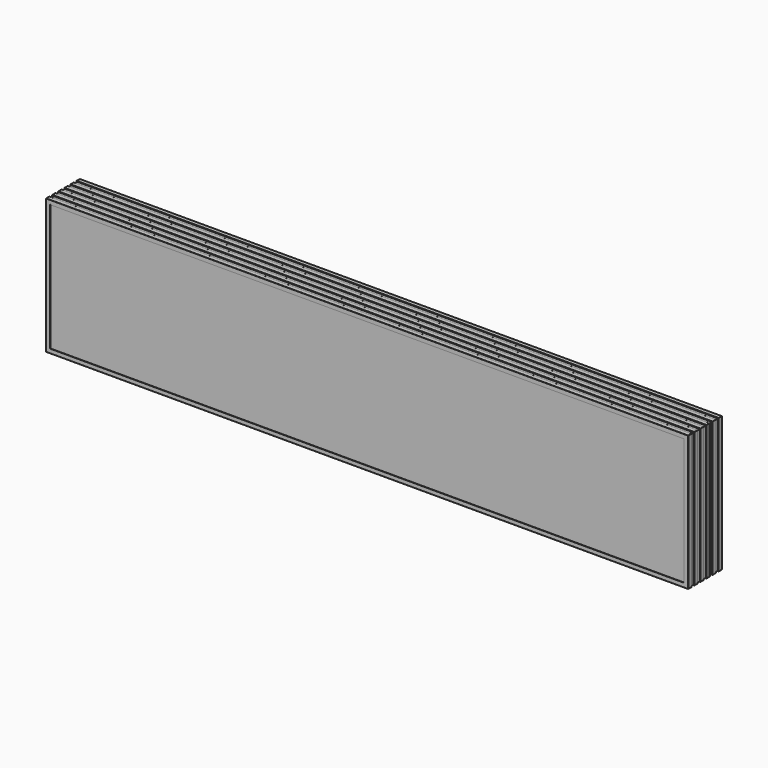
from build123d import *

# Parameters (mm, degrees)
F0_W      = 50
F0_H      = 2720
F1_DEPTH  = 100
F2_W      = 1520
F2_H      = 100
F3_DEPTH  = 320
F2_W_2    = 3000
F2_W_3    = 1220
F4_W      = 1500
F4_H      = 300
F4_W_2    = 2980
F4_W_3    = 1200
F5_DEPTH  = 100.001
F6_W      = 8
F6_H      = 1.5
F7_DEPTH  = 5840.001
F8_W      = 1.5
F8_H      = 8
F9_DEPTH  = 2720.001
F11_W     = 2980
F11_H     = 300
F12_DEPTH = 98
F11_W_2   = 1200
F11_W_3   = 1500
F13_R     = 0.5
F13_2_R   = 0.5
F13_3_R   = 0.5
F13_4_R   = 0.5


# Not quite as in the source:
# - two fillets or chamfers of one size are made in one step


with BuildPart() as f1:
    # F0 (on Front) → F1 (new body)
    with BuildSketch(Plane.XZ):
        with Locations((-1525, -1360)):
            Rectangle(F0_W, F0_H)
    extrude(amount=F1_DEPTH)


with BuildPart() as f1b:
    # F0 (on Front) → F1, piece 2 (new body)
    with BuildSketch(Plane.XZ):
        with Locations((1525, -1360)):
            Rectangle(F0_W, F0_H)
    extrude(amount=F1_DEPTH)


with BuildPart() as f3:
    # F2 (on face) → F3 (new body)
    with BuildSketch(Plane.XY):
        with Locations((-2310, -50)):
            Rectangle(F2_W, F2_H)
    extrude(amount=-F3_DEPTH)


with BuildPart() as f3b:
    # F2 (on face) → F3, piece 2 (new body)
    with BuildSketch(Plane.XY):
        with Locations((0, -50)):
            Rectangle(F2_W_2, F2_H)
    extrude(amount=-F3_DEPTH)


with BuildPart() as f3c:
    # F2 (on face) → F3, piece 3 (new body)
    with BuildSketch(Plane.XY):
        with Locations((2160, -50)):
            Rectangle(F2_W_3, F2_H)
    extrude(amount=-F3_DEPTH)


with BuildPart() as f5_tool:
    # F4 (on face) → F5 (new body, through all)
    with BuildSketch(Plane.XZ.offset(100)):
        with Locations((-2310, -160)):
            Rectangle(F4_W, F4_H)
        with Locations((0, -160)):
            Rectangle(F4_W_2, F4_H)
        with Locations((2160, -160)):
            Rectangle(F4_W_3, F4_H)
    extrude(amount=-F5_DEPTH)


with BuildPart() as f3_1:
    add(f3.part)

    # F5: cut by f5_tool
    add(f5_tool.part, mode=Mode.SUBTRACT)


with BuildPart() as f3b_1:
    add(f3b.part)

    # F5: cut by f5_tool
    add(f5_tool.part, mode=Mode.SUBTRACT)


with BuildPart() as f3c_1:
    add(f3c.part)

    # F5: cut by f5_tool
    add(f5_tool.part, mode=Mode.SUBTRACT)


with BuildPart() as f7_tool:
    # F6 (on face) → F7 (new body, through all)
    with BuildSketch(Plane(origin=(-3070, 0, 0), x_dir=(0, -1, 0), z_dir=(-1, 0, 0))):
        with Locations((14, -0.75)):
            Rectangle(F6_W, F6_H)
        with Locations((32, -0.75)):
            Rectangle(F6_W, F6_H)
        with Locations((50, -0.75)):
            Rectangle(F6_W, F6_H)
        with Locations((68, -0.75)):
            Rectangle(F6_W, F6_H)
        with Locations((86, -0.75)):
            Rectangle(F6_W, F6_H)
        with Locations((86, -319.25)):
            Rectangle(F6_W, F6_H)
        with Locations((68, -319.25)):
            Rectangle(F6_W, F6_H)
        with Locations((14, -319.25)):
            Rectangle(F6_W, F6_H)
        with Locations((32, -319.25)):
            Rectangle(F6_W, F6_H)
        with Locations((50, -319.25)):
            Rectangle(F6_W, F6_H)
    extrude(amount=-F7_DEPTH)


with BuildPart() as f1_1:
    add(f1.part)

    # F7: cut by f7_tool
    add(f7_tool.part, mode=Mode.SUBTRACT)


with BuildPart() as f1b_1:
    add(f1b.part)

    # F7: cut by f7_tool
    add(f7_tool.part, mode=Mode.SUBTRACT)

    # F13
    f13_edges = [f1b_1.edges().sort_by_distance(p)[0] for p in [
        (1525, -90, 0),
        (1525, -100, 0),
        (1525, -72, 0),
        (1525, -82, 0),
        (1525, -54, 0),
        (1525, -64, 0),
        (1525, -36, 0),
        (1525, -46, 0),
        (1525, -18, 0),
        (1525, -28, 0),
        (1525, 0, 0),
        (1525, -10, 0),
    ]]
    fillet(f13_edges, radius=F13_R)


with BuildPart() as f3_2:
    add(f3_1.part)

    # F7: cut by f7_tool
    add(f7_tool.part, mode=Mode.SUBTRACT)

    # F8 (on face) → F9 (cut, through all)
    with BuildSketch(Plane.XY):
        with Locations((-3069.25, -86)):
            Rectangle(F8_W, F8_H)
        with Locations((-3069.25, -68)):
            Rectangle(F8_W, F8_H)
        with Locations((-3069.25, -50)):
            Rectangle(F8_W, F8_H)
        with Locations((-3069.25, -32)):
            Rectangle(F8_W, F8_H)
        with Locations((-3069.25, -14)):
            Rectangle(F8_W, F8_H)
        with Locations((3069.25, -68)):
            Rectangle(F8_W, F8_H)
        with Locations((3069.25, -32)):
            Rectangle(F8_W, F8_H)
        with Locations((3069.25, -86)):
            Rectangle(F8_W, F8_H)
        with Locations((3069.25, -50)):
            Rectangle(F8_W, F8_H)
        with Locations((3069.25, -14)):
            Rectangle(F8_W, F8_H)
        with Locations((-1550.75, -86)):
            Rectangle(F8_W, F8_H)
        with Locations((-1550.75, -68)):
            Rectangle(F8_W, F8_H)
        with Locations((-1550.75, -50)):
            Rectangle(F8_W, F8_H)
        with Locations((-1550.75, -32)):
            Rectangle(F8_W, F8_H)
        with Locations((-1550.75, -14)):
            Rectangle(F8_W, F8_H)
    extrude(amount=-F9_DEPTH, mode=Mode.SUBTRACT)

    # F13#2
    f13_2_edges = [f3_2.edges().sort_by_distance(p)[0] for p in [
        (-1550, -5, -320),
        (-1550, -23, -320),
        (-1550, -41, -320),
        (-1550, -59, -320),
        (-1550, -77, -320),
        (-1550, -95, -320),
        (-3070, -95, -320),
        (-3068.5, -86, -318.5),
        (-3070, -77, -320),
        (-3068.5, -68, -318.5),
        (-3070, -59, -320),
        (-3068.5, -50, -318.5),
        (-3070, -41, -320),
        (-3068.5, -32, -318.5),
        (-3070, -23, -320),
        (-3068.5, -14, -318.5),
        (-3070, -5, -320),
        (-3070, -95, 0),
        (-3068.5, -86, -1.5),
        (-3070, -77, 0),
        (-3068.5, -68, -1.5),
        (-3070, -59, 0),
        (-3068.5, -50, -1.5),
        (-3070, -41, 0),
        (-3068.5, -32, -1.5),
        (-3070, -23, 0),
        (-3068.5, -14, -1.5),
        (-3070, -5, 0),
        (-1550, -95, 0),
        (-1550, -77, 0),
        (-1550, -59, 0),
        (-1550, -41, 0),
        (-1550, -23, 0),
        (-1550, -5, 0),
        (-1551.5, -32, -1.5),
        (-1551.5, -14, -1.5),
        (-1551.5, -50, -1.5),
        (-1551.5, -68, -1.5),
        (-1551.5, -86, -1.5),
        (-3070, -100, -160),
        (-2310, -100, 0),
        (-2310, -100, -320),
        (-1550, -100, -160),
        (-1550, 0, -160),
        (-2310, 0, 0),
        (-2310, 0, -320),
        (-3070, 0, -160),
        (-3070, -10, -160),
        (-1550, -10, -160),
        (-2310, -10, -320),
        (-2310, -10, 0),
        (-1550, -18, -160),
        (-2310, -18, 0),
        (-3070, -18, -160),
        (-2310, -18, -320),
        (-2310, -28, -320),
        (-1550, -28, -160),
        (-3070, -28, -160),
        (-2310, -28, 0),
        (-1550, -36, -160),
        (-2310, -36, 0),
        (-3070, -36, -160),
        (-2310, -36, -320),
        (-2310, -46, -320),
        (-2310, -46, 0),
        (-1550, -46, -160),
        (-3070, -46, -160),
        (-3070, -54, -160),
        (-2310, -54, -320),
        (-1550, -54, -160),
        (-2310, -54, 0),
        (-2310, -64, 0),
        (-3070, -64, -160),
        (-1550, -64, -160),
        (-2310, -64, -320),
        (-3070, -72, -160),
        (-2310, -72, -320),
        (-1550, -72, -160),
        (-2310, -72, 0),
        (-2310, -82, 0),
        (-3070, -82, -160),
        (-1550, -82, -160),
        (-2310, -82, -320),
        (-3070, -90, -160),
        (-2310, -90, -320),
        (-1550, -90, -160),
        (-2310, -90, 0),
    ]]
    fillet(f13_2_edges, radius=F13_2_R)


with BuildPart() as f3b_2:
    add(f3b_1.part)

    # F7: cut by f7_tool
    add(f7_tool.part, mode=Mode.SUBTRACT)

    # F13#3
    f13_3_edges = [f3b_2.edges().sort_by_distance(p)[0] for p in [
        (1500, -95, 0),
        (1500, -77, 0),
        (1500, -59, 0),
        (1500, -41, 0),
        (1500, -23, 0),
        (1500, -5, 0),
        (1500, -86, -1.5),
        (1500, -68, -1.5),
        (1500, -50, -1.5),
        (1500, -32, -1.5),
        (1500, -14, -1.5),
        (1500, -95, -320),
        (1500, -86, -318.5),
        (1500, -77, -320),
        (1500, -68, -318.5),
        (1500, -59, -320),
        (1500, -50, -318.5),
        (1500, -41, -320),
        (1500, -32, -318.5),
        (1500, -23, -320),
        (1500, -14, -318.5),
        (1500, -5, -320),
        (-1500, -5, -320),
        (-1500, -23, -320),
        (-1500, -32, -318.5),
        (-1500, -41, -320),
        (-1500, -50, -318.5),
        (-1500, -59, -320),
        (-1500, -68, -318.5),
        (-1500, -77, -320),
        (-1500, -86, -318.5),
        (-1500, -95, -320),
        (-1500, -14, -318.5),
        (-1500, -95, 0),
        (-1500, -77, 0),
        (-1500, -59, 0),
        (-1500, -68, -1.5),
        (-1500, -86, -1.5),
        (-1500, -50, -1.5),
        (-1500, -41, 0),
        (-1500, -32, -1.5),
        (-1500, -23, 0),
        (-1500, -14, -1.5),
        (-1500, -5, 0),
    ]]
    fillet(f13_3_edges, radius=F13_3_R)


with BuildPart() as f3c_2:
    add(f3c_1.part)

    # F7: cut by f7_tool
    add(f7_tool.part, mode=Mode.SUBTRACT)

    # F13#4
    f13_4_edges = [f3c_2.edges().sort_by_distance(p)[0] for p in [
        (2770, -5, 0),
        (2770, -23, 0),
        (2770, -41, 0),
        (2770, -59, 0),
        (2770, -77, 0),
        (2770, -95, 0),
        (1550, -5, 0),
        (1550, -23, 0),
        (1550, -41, 0),
        (1550, -59, 0),
        (1550, -95, 0),
        (1550, -77, 0),
        (1550, -86, -1.5),
        (1550, -68, -1.5),
        (1550, -50, -1.5),
        (1550, -32, -1.5),
        (1550, -14, -1.5),
        (2770, -5, -320),
        (2770, -23, -320),
        (2770, -41, -320),
        (2770, -59, -320),
        (2770, -77, -320),
        (2770, -95, -320),
        (1550, -5, -320),
        (1550, -14, -318.5),
        (1550, -23, -320),
        (1550, -32, -318.5),
        (1550, -41, -320),
        (1550, -50, -318.5),
        (1550, -59, -320),
        (1550, -68, -318.5),
        (1550, -77, -320),
        (1550, -86, -318.5),
        (1550, -95, -320),
    ]]
    fillet(f13_4_edges, radius=F13_4_R)


with BuildPart() as f12:
    # F11 (on offset) → F12 (new body, through all)
    with BuildSketch(Plane(origin=(0, -1, 0), x_dir=(-1, 0, 0), z_dir=(0, 1, 0))):
        with Locations((0, -160)):
            Rectangle(F11_W, F11_H)
    extrude(amount=-F12_DEPTH)


with BuildPart() as f12b:
    # F11 (on offset) → F12, piece 2 (new body, through all)
    with BuildSketch(Plane(origin=(0, -1, 0), x_dir=(-1, 0, 0), z_dir=(0, 1, 0))):
        with Locations((-2160, -160)):
            Rectangle(F11_W_2, F11_H)
    extrude(amount=-F12_DEPTH)


with BuildPart() as f12c:
    # F11 (on offset) → F12, piece 3 (new body, through all)
    with BuildSketch(Plane(origin=(0, -1, 0), x_dir=(-1, 0, 0), z_dir=(0, 1, 0))):
        with Locations((2310, -160)):
            Rectangle(F11_W_3, F11_H)
    extrude(amount=-F12_DEPTH)


solid = Compound([f3_2.part, f12c.part])
